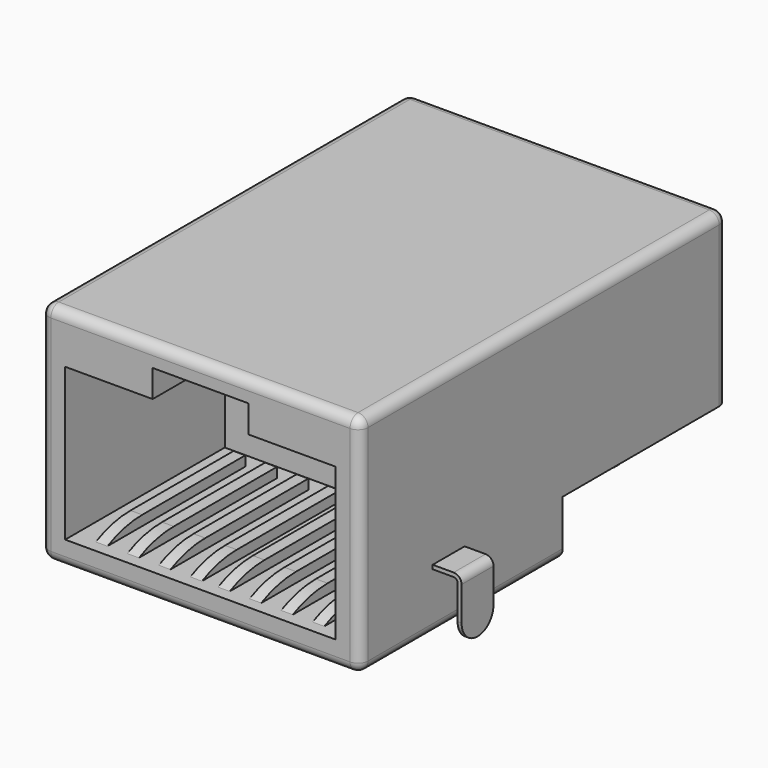
from build123d import *

# Parameters (mm, degrees)
F0_W           = 16
F0_H           = 23
F1_DEPTH       = 8.51
F2_W           = 16
F2_H           = 12.7
F3_DEPTH       = 2.79
F4_R           = 0.5
F5_R           = 0.8
F6_DEPTH       = 2.5
F7_SIZE        = 0.3
F9_DEPTH       = 10
F10_W          = 0.5874776107
F10_H          = 8.6386585608
F11_DEPTH      = 0.5
F12_T1_DEPTH   = 11.4847249695
F12_2_T1_DEPTH = 11.4847249695
F12_3_T1_DEPTH = 11.4847249695
F12_4_T1_DEPTH = 11.4847249695
F12_5_T1_DEPTH = 11.4847249695
F12_6_T1_DEPTH = 11.4847249695
F12_7_T1_DEPTH = 11.4847249695
F12_8_T1_DEPTH = 11.4847249695
F13_W          = 0.45
F13_H          = 0.35
F14_DEPTH      = 2.79
F17_DEPTH      = 1
F17_DEPTH_BACK = 1
F18_R          = 0.99999


# Not quite as in the source:
# - a fillet or chamfer that OpenCascade refuses, or shapes differently, is made with other operations: its cross-section is extruded or revolved along the edge and cut away or added
# - a fillet or chamfer is up to 0.001 mm smaller than in the source, because OpenCascade refuses the exact size


with BuildPart() as f1:
    # F0 (on Top) → F1 (new body)
    with BuildSketch(Plane.XY):
        Rectangle(F0_W, F0_H)
    extrude(amount=F1_DEPTH)

    # F2 (on face) → F3 (join)
    with BuildSketch(Plane(origin=(0, 0, 0), x_dir=(1, 0, 0), z_dir=(0, 0, -1))):
        with Locations((0, 5.15)):
            Rectangle(F2_W, F2_H)
    extrude(amount=F3_DEPTH)

    # F4
    f4_edges = [f1.edges().sort_by_distance(p)[0] for p in [
        (-8, -11.5, 2.86),
        (8, -11.5, 2.86),
        (8, 11.5, 4.255),
        (-8, 11.5, 4.255),
        (0, -11.5, 8.51),
        (-8, 0, 8.51),
        (0, 11.5, 8.51),
        (8, 0, 8.51),
        (0, -11.5, -2.79),
        (-8, -5.15, -2.79),
        (8, -5.15, -2.79),
    ]]
    fillet(f4_edges, radius=F4_R)

    # F5 (on face) → F6 (join)
    with BuildSketch(Plane(origin=(0, 0, 0), x_dir=(1, 0, 0), z_dir=(0, 0, -1))):
        with Locations((4.5, -3.3)):
            Circle(F5_R)
        with Locations((-4.5, -3.3)):
            Circle(F5_R)
    extrude(amount=F6_DEPTH)

    # F7
    f7_edges = [f1.edges().sort_by_distance(p)[0] for p in [
        (3.7, 3.3, -2.5),
        (-5.3, 3.3, -2.5),
    ]]
    chamfer(f7_edges, length=F7_SIZE)

    # F8 (on face) → F9 (cut)
    with BuildSketch(Plane.XZ.offset(11.5)):
        Polygon((2.3968075402, 7.4636251666), (0, 7.4636251666), (-2.3968075402, 7.4636251666), (-2.3968075402, 6.0898447409), (-6.7812129855, 6.0898447409), (-6.7812129855, -1.5390195185), (0, -1.5390195185), (6.7812129855, -1.5390195185), (6.7812129855, 6.0898447409), (2.3968075402, 6.0898447409), align=None)
    extrude(amount=-F9_DEPTH, mode=Mode.SUBTRACT)

    # F13 (on face) → F14 (join)
    with BuildSketch(Plane(origin=(0, 0, 0), x_dir=(1, 0, 0), z_dir=(0, 0, -1))):
        with Locations((4.445, -8.76)):
            Rectangle(F13_W, F13_H)
        with Locations((1.905, -8.76)):
            Rectangle(F13_W, F13_H)
        with Locations((-0.635, -8.76)):
            Rectangle(F13_W, F13_H)
        with Locations((-3.175, -8.76)):
            Rectangle(F13_W, F13_H)
        with Locations((3.175, -6.22)):
            Rectangle(F13_W, F13_H)
        with Locations((0.635, -6.22)):
            Rectangle(F13_W, F13_H)
        with Locations((-1.905, -6.22)):
            Rectangle(F13_W, F13_H)
        with Locations((-4.445, -6.22)):
            Rectangle(F13_W, F13_H)
    extrude(amount=F14_DEPTH)

    # F16 (on offset) → F17 (join, two sides)
    with BuildSketch(Plane.XZ.offset(5.95)) as f17_sk:
        with BuildLine():
            Line((9.05, 0.31), (8, 0.31))
            Line((8, 0.31), (8, 0.11))
            Line((8, 0.11), (9.05, 0.11))
            ThreePointArc((9.05, 0.11), (9.1914213562, 0.0514213562), (9.25, -0.09))
            Line((9.25, -0.09), (9.25, -2.79))
            Line((9.25, -2.79), (9.45, -2.79))
            Line((9.45, -2.79), (9.45, -0.09))
            ThreePointArc((9.45, -0.09), (9.3328427125, 0.1928427125), (9.05, 0.31))
        make_face()
        with BuildLine():
            Line((-9.45, -2.79), (-9.25, -2.79))
            Line((-9.25, -2.79), (-9.25, -0.09))
            ThreePointArc((-9.25, -0.09), (-9.1914213562, 0.0514213562), (-9.05, 0.11))
            Line((-9.05, 0.11), (-8, 0.11))
            Line((-8, 0.11), (-8, 0.31))
            Line((-8, 0.31), (-9.05, 0.31))
            ThreePointArc((-9.05, 0.31), (-9.3328427125, 0.1928427125), (-9.45, -0.09))
            Line((-9.45, -0.09), (-9.45, -2.79))
        make_face()
    extrude(amount=F17_DEPTH)
    extrude(f17_sk.sketch, amount=-F17_DEPTH_BACK)

    # F18 (radius 1 in the source; OpenCascade refuses exactly that, so slightly less here)
    f18_edges = [f1.edges().sort_by_distance(p)[0] for p in [
        (9.35, -6.95, -2.79),
        (9.35, -4.95, -2.79),
        (-9.35, -6.95, -2.79),
        (-9.35, -4.95, -2.79),
    ]]
    fillet(f18_edges, radius=F18_R)


with BuildPart() as f11:
    # F10 (on face) → F11 (new body)
    with BuildSketch(Plane.XY.offset(-1.5390195185)):
        with Locations((0.6958528975, -6.5825465135)):
            Rectangle(F10_W, F10_H)
    extrude(amount=F11_DEPTH)

    # F12: fillet of radius 5 on 1 edges, made by hand

    # F12_s2 → F12_t1 (cut)
    with BuildSketch(Plane.YZ.offset(-5.0465095873)):
        with BuildLine():
            ThreePointArc((-10.9018757939, -1.5390195185), (-9.8404603109, -1.1656223461), (-8.7224263222, -1.0390195185))
            Line((-8.7224263222, -1.0390195185), (-10.9018757939, -1.0390195185))
            Line((-10.9018757939, -1.0390195185), (-10.9018757939, -1.5390195185))
        make_face()
    extrude(amount=F12_T1_DEPTH, mode=Mode.SUBTRACT)


with BuildPart() as f11b:
    # F10 (on face) → F11, piece 2 (new body)
    with BuildSketch(Plane.XY.offset(-1.5390195185)):
        with Locations((2.2758528975, -6.5825465135)):
            Rectangle(F10_W, F10_H)
    extrude(amount=F11_DEPTH)

    # F12#2: fillet of radius 5 on 1 edges, made by hand

    # F12_2_s2 → F12_2_t1 (cut)
    with BuildSketch(Plane.YZ.offset(-3.4665095873)):
        with BuildLine():
            ThreePointArc((-10.9018757939, -1.5390195185), (-9.8404603109, -1.1656223461), (-8.7224263222, -1.0390195185))
            Line((-8.7224263222, -1.0390195185), (-10.9018757939, -1.0390195185))
            Line((-10.9018757939, -1.0390195185), (-10.9018757939, -1.5390195185))
        make_face()
    extrude(amount=F12_2_T1_DEPTH, mode=Mode.SUBTRACT)


with BuildPart() as f11c:
    # F10 (on face) → F11, piece 3 (new body)
    with BuildSketch(Plane.XY.offset(-1.5390195185)):
        with Locations((3.8558528975, -6.5825465135)):
            Rectangle(F10_W, F10_H)
    extrude(amount=F11_DEPTH)

    # F12#3: fillet of radius 5 on 1 edges, made by hand

    # F12_3_s2 → F12_3_t1 (cut)
    with BuildSketch(Plane.YZ.offset(-1.8865095873)):
        with BuildLine():
            ThreePointArc((-10.9018757939, -1.5390195185), (-9.8404603109, -1.1656223461), (-8.7224263222, -1.0390195185))
            Line((-8.7224263222, -1.0390195185), (-10.9018757939, -1.0390195185))
            Line((-10.9018757939, -1.0390195185), (-10.9018757939, -1.5390195185))
        make_face()
    extrude(amount=F12_3_T1_DEPTH, mode=Mode.SUBTRACT)


with BuildPart() as f11d:
    # F10 (on face) → F11, piece 4 (new body)
    with BuildSketch(Plane.XY.offset(-1.5390195185)):
        with Locations((5.4358528975, -6.5825465135)):
            Rectangle(F10_W, F10_H)
    extrude(amount=F11_DEPTH)

    # F12#4: fillet of radius 5 on 1 edges, made by hand

    # F12_4_s2 → F12_4_t1 (cut)
    with BuildSketch(Plane.YZ.offset(-0.3065095873)):
        with BuildLine():
            ThreePointArc((-10.9018757939, -1.5390195185), (-9.8404603109, -1.1656223461), (-8.7224263222, -1.0390195185))
            Line((-8.7224263222, -1.0390195185), (-10.9018757939, -1.0390195185))
            Line((-10.9018757939, -1.0390195185), (-10.9018757939, -1.5390195185))
        make_face()
    extrude(amount=F12_4_T1_DEPTH, mode=Mode.SUBTRACT)


with BuildPart() as f11e:
    # F10 (on face) → F11, piece 5 (new body)
    with BuildSketch(Plane.XY.offset(-1.5390195185)):
        with Locations((-0.6958528975, -6.5825465135)):
            Rectangle(F10_W, F10_H)
    extrude(amount=F11_DEPTH)

    # F12#5: fillet of radius 5 on 1 edges, made by hand

    # F12_5_s2 → F12_5_t1 (cut)
    with BuildSketch(Plane.YZ.offset(-6.4382153822)):
        with BuildLine():
            ThreePointArc((-10.9018757939, -1.5390195185), (-9.8404603109, -1.1656223461), (-8.7224263222, -1.0390195185))
            Line((-8.7224263222, -1.0390195185), (-10.9018757939, -1.0390195185))
            Line((-10.9018757939, -1.0390195185), (-10.9018757939, -1.5390195185))
        make_face()
    extrude(amount=F12_5_T1_DEPTH, mode=Mode.SUBTRACT)


with BuildPart() as f11f:
    # F10 (on face) → F11, piece 6 (new body)
    with BuildSketch(Plane.XY.offset(-1.5390195185)):
        with Locations((-3.8558528975, -6.5825465135)):
            Rectangle(F10_W, F10_H)
    extrude(amount=F11_DEPTH)

    # F12#6: fillet of radius 5 on 1 edges, made by hand

    # F12_6_s2 → F12_6_t1 (cut)
    with BuildSketch(Plane.YZ.offset(-9.5982153822)):
        with BuildLine():
            ThreePointArc((-10.9018757939, -1.5390195185), (-9.8404603109, -1.1656223461), (-8.7224263222, -1.0390195185))
            Line((-8.7224263222, -1.0390195185), (-10.9018757939, -1.0390195185))
            Line((-10.9018757939, -1.0390195185), (-10.9018757939, -1.5390195185))
        make_face()
    extrude(amount=F12_6_T1_DEPTH, mode=Mode.SUBTRACT)


with BuildPart() as f11g:
    # F10 (on face) → F11, piece 7 (new body)
    with BuildSketch(Plane.XY.offset(-1.5390195185)):
        with Locations((-2.2758528975, -6.5825465135)):
            Rectangle(F10_W, F10_H)
    extrude(amount=F11_DEPTH)

    # F12#7: fillet of radius 5 on 1 edges, made by hand

    # F12_7_s2 → F12_7_t1 (cut)
    with BuildSketch(Plane.YZ.offset(-8.0182153822)):
        with BuildLine():
            ThreePointArc((-10.9018757939, -1.5390195185), (-9.8404603109, -1.1656223461), (-8.7224263222, -1.0390195185))
            Line((-8.7224263222, -1.0390195185), (-10.9018757939, -1.0390195185))
            Line((-10.9018757939, -1.0390195185), (-10.9018757939, -1.5390195185))
        make_face()
    extrude(amount=F12_7_T1_DEPTH, mode=Mode.SUBTRACT)


with BuildPart() as f11h:
    # F10 (on face) → F11, piece 8 (new body)
    with BuildSketch(Plane.XY.offset(-1.5390195185)):
        with Locations((-5.4358528975, -6.5825465135)):
            Rectangle(F10_W, F10_H)
    extrude(amount=F11_DEPTH)

    # F12#8: fillet of radius 5 on 1 edges, made by hand

    # F12_8_s2 → F12_8_t1 (cut)
    with BuildSketch(Plane.YZ.offset(-11.1782153822)):
        with BuildLine():
            ThreePointArc((-10.9018757939, -1.5390195185), (-9.8404603109, -1.1656223461), (-8.7224263222, -1.0390195185))
            Line((-8.7224263222, -1.0390195185), (-10.9018757939, -1.0390195185))
            Line((-10.9018757939, -1.0390195185), (-10.9018757939, -1.5390195185))
        make_face()
    extrude(amount=F12_8_T1_DEPTH, mode=Mode.SUBTRACT)


solid = Compound([f1.part, f11.part, f11b.part, f11c.part, f11d.part, f11e.part, f11f.part, f11g.part, f11h.part])
